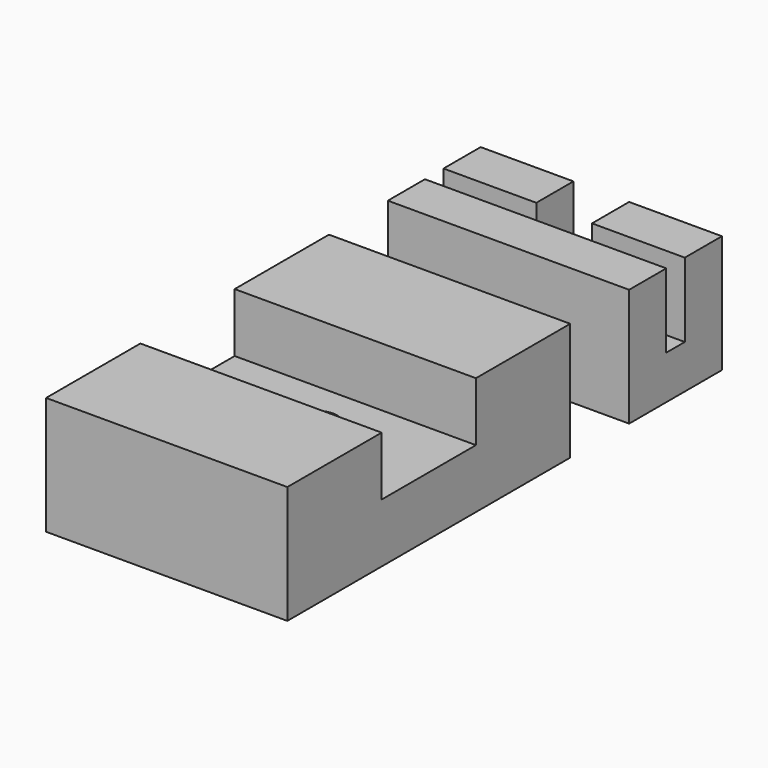
from build123d import *

# Parameters (mm, degrees)
F0_W     = 26
F0_H     = 5
F0_W_2   = 10
F0_W_3   = 6
F1_DEPTH = 12.7
F2_DEPTH = 8
F3_W     = 26
F3_H     = 12.7
F4_DEPTH = 12.7
F5_DEPTH = 6.35
F6_D     = 4.5


# Not quite as in the source:
# - a length typed as a fraction of an inch, garbled in the dataset ("3 / 203.2 mm" for 3/8 in), is restored


with BuildPart() as f1:
    # F0 (on Top) → F1 (new body)
    with BuildSketch(Plane.XY):
        with Locations((0, -3.75)):
            Rectangle(F0_W, F0_H)
        Polygon((-13, -1.25), (13, -1.25), (13, 1.25), (3, 1.25), (-3, 1.25), (-13, 1.25), align=None)
        with Locations((8, 3.75)):
            Rectangle(F0_W_2, F0_H)
        with Locations((-8, 3.75)):
            Rectangle(F0_W_2, F0_H)
        with Locations((0, 3.75)):
            Rectangle(F0_W_3, F0_H)
    extrude(amount=-F1_DEPTH)

    # F0 (on Top) → F2 (cut)
    with BuildSketch(Plane.XY):
        with Locations((0, 3.75)):
            Rectangle(F0_W_3, F0_H)
        Polygon((-13, -1.25), (13, -1.25), (13, 1.25), (3, 1.25), (-3, 1.25), (-13, 1.25), align=None)
    extrude(amount=-F2_DEPTH, mode=Mode.SUBTRACT)


with BuildPart() as f4:
    # F3 (on Top) → F4 (new body)
    with BuildSketch(Plane.XY):
        with Locations((0, -20.533909303)):
            Rectangle(F3_W, F3_H)
        with Locations((0, -33.233909303)):
            Rectangle(F3_W, F3_H)
        with Locations((0, -45.933909303)):
            Rectangle(F3_W, F3_H)
    extrude(amount=-F4_DEPTH)

    # F3 (on Top) → F5 (cut)
    with BuildSketch(Plane.XY):
        with Locations((0, -33.233909303)):
            Rectangle(F3_W, F3_H)
    extrude(amount=-F5_DEPTH, mode=Mode.SUBTRACT)

    # F6 (through all)
    with Locations(Plane.XY):
        with Locations((0, -32.133909303)):
            Hole(F6_D / 2)


solid = Compound([f1.part, f4.part])
